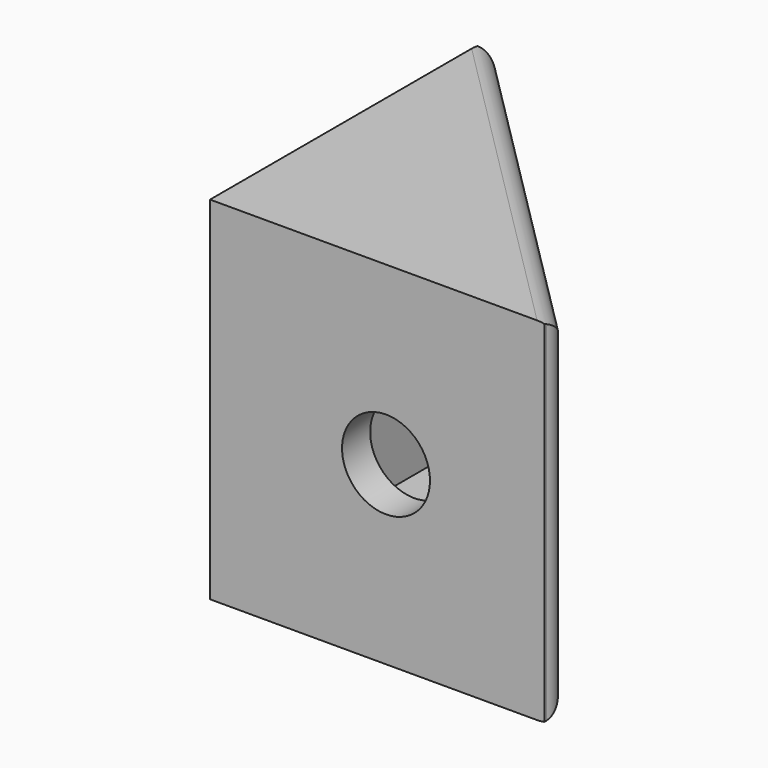
from build123d import *

# Parameters (mm, degrees)
F0_DEPTH    = 20
F1_T        = -2
F4_D        = 5
F4_ON_F2_D  = 5
F5_SIZE     = 1
F7_T1_DEPTH = 31.2842712475
F7_T3_DEPTH = 23.3408931896


# Not quite as in the source:
# - a fillet or chamfer that OpenCascade refuses, or shapes differently, is made with other operations: its cross-section is extruded or revolved along the edge and cut away or added


with BuildPart() as f0:
    # F6 (on Top) → F0 (new body)
    with BuildSketch(Plane.XY):
        Polygon((-10, -10), (10, -10), (-10, 10), align=None)
    extrude(amount=F0_DEPTH)

    # F1
    f1_openings = [f0.faces().sort_by_distance(p)[0] for p in [
        (0, 0, 10),
    ]]
    offset(amount=F1_T, openings=f1_openings)

    # F4 (through all)
    with Locations(Plane(origin=(0, -8, 0), x_dir=(-1, 0, 0), z_dir=(0, 1, 0))):
        with Locations((0, 10)):
            Hole(F4_D / 2)

    # F4 on F2 (through all)
    with Locations(Plane.YZ.offset(-8)):
        with Locations((0, 10)):
            Hole(F4_ON_F2_D / 2)

    # F5
    f5_edges = [f0.edges().sort_by_distance(p)[0] for p in [
        (-10, 10, 10),
        (10, -10, 10),
    ]]
    chamfer(f5_edges, length=F5_SIZE)

    # F7: fillet of radius 1 on 4 edges, made by hand

    # F7_s2 → F7_t1 (cut)
    with BuildSketch(Plane(origin=(11.0606601718, -11.0606601718, 0), x_dir=(0, 0, 1), z_dir=(-0.7071067812, 0.7071067812, 0))):
        with BuildLine():
            ThreePointArc((0, -1), (0.2928932188, -0.2928932188), (1, 0))
            Line((1, 0), (0, 0))
            Line((0, 0), (0, -1))
        make_face()
        with BuildLine():
            ThreePointArc((20, -1), (19.7071067812, -0.2928932188), (19, 0))
            Line((19, 0), (20, 0))
            Line((20, 0), (20, -1))
        make_face()
    extrude(amount=F7_T1_DEPTH, mode=Mode.SUBTRACT)

    # F7_s4 → F7_t3 (cut)
    with BuildSketch(Plane.XY.offset(-1.6704465948)):
        with BuildLine():
            ThreePointArc((9.0371923242, -9.9102097864), (9.0940980721, -9.3324360321), (8.8204195729, -8.8204195729))
            Line((8.8204195729, -8.8204195729), (9.2928932188, -9.2928932188))
            Line((9.2928932188, -9.2928932188), (9.0371923242, -9.9102097864))
        make_face()
        with BuildLine():
            ThreePointArc((-8.8204195729, 8.8204195729), (-9.3324360321, 9.0940980721), (-9.9102097864, 9.0371923242))
            Line((-9.9102097864, 9.0371923242), (-9.2928932188, 9.2928932188))
            Line((-9.2928932188, 9.2928932188), (-8.8204195729, 8.8204195729))
        make_face()
    extrude(amount=F7_T3_DEPTH, mode=Mode.SUBTRACT)


solid = f0.part
